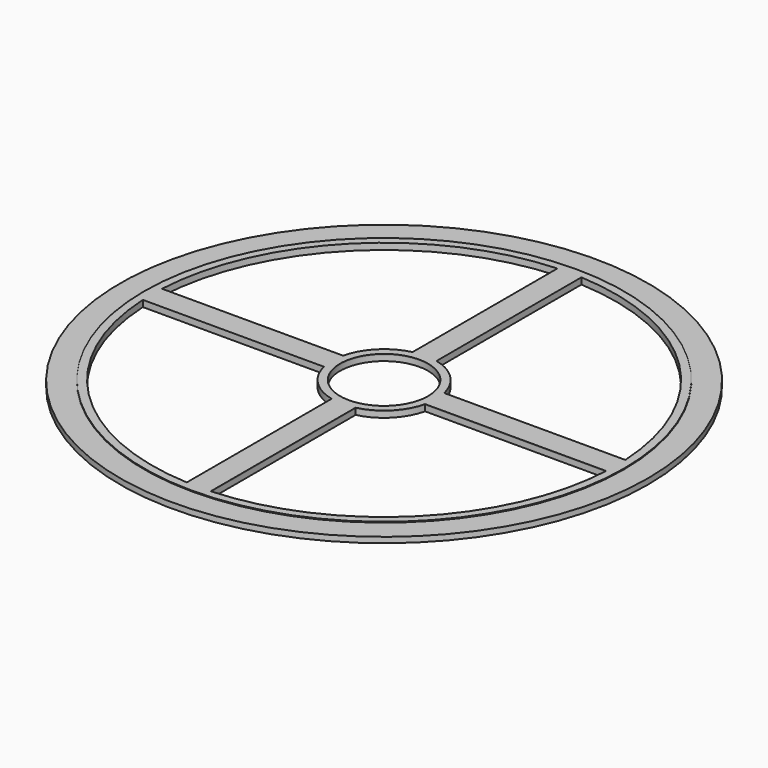
from build123d import *

# Parameters (mm, degrees)
F0_R     = 30
F1_DEPTH = 0.1
F2_R     = 5.5
F3_DEPTH = 0.1
F5_DEPTH = 0.1
F6_R     = 33
F6_R_2   = 30
F6_R_3   = 5.5
F7_DEPTH = 0.7


with BuildPart() as f1:
    # F0 (on Top) → F1 (new body)
    with BuildSketch(Plane.XY):
        Circle(F0_R)
    extrude(amount=F1_DEPTH)

    # F2 (on face) → F3 (cut, through all)
    with BuildSketch(Plane.XY.offset(0.1)):
        Circle(F2_R)
    extrude(amount=-F3_DEPTH, mode=Mode.SUBTRACT)

    # F4 (on face) → F5 (cut, through all)
    with BuildSketch(Plane.XY.offset(0.1)):
        with BuildLine():
            Line((6.3245553203, 1.5), (28.9611809151, 1.5))
            ThreePointArc((28.9611809151, 1.5), (20.5060966544, 20.5060966544), (1.5, 28.9611809151))
            Line((1.5, 28.9611809151), (1.5, 6.3245553203))
            ThreePointArc((1.5, 6.3245553203), (4.5961940777, 4.5961940777), (6.3245553203, 1.5))
        make_face()
        with BuildLine():
            Line((-1.5, 6.3245553203), (-1.5, 28.9611809151))
            ThreePointArc((-1.5, 28.9611809151), (-20.5060966544, 20.5060966544), (-28.9611809151, 1.5))
            Line((-28.9611809151, 1.5), (-6.3245553203, 1.5))
            ThreePointArc((-6.3245553203, 1.5), (-4.5961940777, 4.5961940777), (-1.5, 6.3245553203))
        make_face()
        with BuildLine():
            ThreePointArc((-28.9611809151, -1.5), (-20.5060966544, -20.5060966544), (-1.5, -28.9611809151))
            Line((-1.5, -28.9611809151), (-1.5, -6.3245553203))
            ThreePointArc((-1.5, -6.3245553203), (-4.5961940777, -4.5961940777), (-6.3245553203, -1.5))
            Line((-6.3245553203, -1.5), (-28.9611809151, -1.5))
        make_face()
        with BuildLine():
            ThreePointArc((1.5, -28.9611809151), (20.5060966544, -20.5060966544), (28.9611809151, -1.5))
            Line((28.9611809151, -1.5), (6.3245553203, -1.5))
            ThreePointArc((6.3245553203, -1.5), (4.5961940777, -4.5961940777), (1.5, -6.3245553203))
            Line((1.5, -6.3245553203), (1.5, -28.9611809151))
        make_face()
    extrude(amount=-F5_DEPTH, mode=Mode.SUBTRACT)

    # F6 (on face) → F7 (join)
    with BuildSketch(Plane(origin=(0, 0, 0), x_dir=(1, 0, 0), z_dir=(0, 0, -1))):
        Circle(F6_R)
        Circle(F6_R_2, mode=Mode.SUBTRACT)
        Circle(F6_R_2)
        with BuildLine():
            Line((-1.5, -6.3245553203), (-1.5, -28.9611809151))
            ThreePointArc((-1.5, -28.9611809151), (-20.5060966544, -20.5060966544), (-28.9611809151, -1.5))
            Line((-28.9611809151, -1.5), (-6.3245553203, -1.5))
            ThreePointArc((-6.3245553203, -1.5), (-4.5961940777, -4.5961940777), (-1.5, -6.3245553203))
        make_face(mode=Mode.SUBTRACT)
        with BuildLine():
            ThreePointArc((28.9611809151, -1.5), (20.5060966544, -20.5060966544), (1.5, -28.9611809151))
            Line((1.5, -28.9611809151), (1.5, -6.3245553203))
            ThreePointArc((1.5, -6.3245553203), (4.5961940777, -4.5961940777), (6.3245553203, -1.5))
            Line((6.3245553203, -1.5), (28.9611809151, -1.5))
        make_face(mode=Mode.SUBTRACT)
        with BuildLine():
            ThreePointArc((-1.5, 6.3245553203), (-4.5961940777, 4.5961940777), (-6.3245553203, 1.5))
            Line((-6.3245553203, 1.5), (-28.9611809151, 1.5))
            ThreePointArc((-28.9611809151, 1.5), (-20.5060966544, 20.5060966544), (-1.5, 28.9611809151))
            Line((-1.5, 28.9611809151), (-1.5, 6.3245553203))
        make_face(mode=Mode.SUBTRACT)
        Circle(F6_R_3, mode=Mode.SUBTRACT)
        with BuildLine():
            Line((1.5, 6.3245553203), (1.5, 28.9611809151))
            ThreePointArc((1.5, 28.9611809151), (20.5060966544, 20.5060966544), (28.9611809151, 1.5))
            Line((28.9611809151, 1.5), (6.3245553203, 1.5))
            ThreePointArc((6.3245553203, 1.5), (4.5961940777, 4.5961940777), (1.5, 6.3245553203))
        make_face(mode=Mode.SUBTRACT)
    extrude(amount=F7_DEPTH)


solid = f1.part
